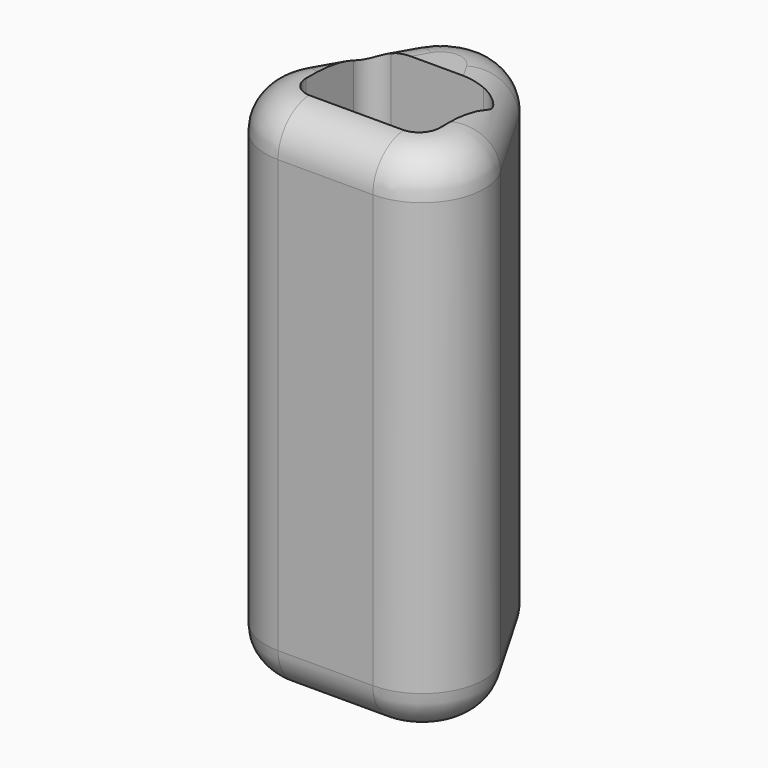
from build123d import *

# Parameters (mm, degrees)
F1_DEPTH     = 25
F2_T1_DEPTH  = 4.6076951546
F2_T3_DEPTH  = 4.6076951546
F2_T5_DEPTH  = 4.6076951546
F2_T8_ANGLE  = 120
F2_T10_ANGLE = 120
F2_T12_ANGLE = 120
F2_T14_ANGLE = 120
F2_T16_ANGLE = 120
F2_T18_ANGLE = 120


# Not quite as in the source:
# - a fillet or chamfer that OpenCascade refuses, or shapes differently, is made with other operations: its cross-section is extruded or revolved along the edge and cut away or added


with BuildPart() as f1:
    # F0 (on Top) → F1 (new body)
    with BuildSketch(Plane.XY):
        with BuildLine():
            Line((-2.3038475773, -4.3301270189), (2.3038475773, -4.3301270189))
            ThreePointArc((2.3038475773, -4.3301270189), (4.9019237886, -2.8301270189), (4.9019237886, 0.1698729811))
            Line((4.9019237886, 0.1698729811), (2.5980762114, 4.1602540378))
            ThreePointArc((2.5980762114, 4.1602540378), (0, 5.6602540378), (-2.5980762114, 4.1602540378))
            Line((-2.5980762114, 4.1602540378), (-4.9019237886, 0.1698729811))
            ThreePointArc((-4.9019237886, 0.1698729811), (-4.9019237886, -2.8301270189), (-2.3038475773, -4.3301270189))
        make_face()
        with BuildLine():
            ThreePointArc((3.25, -1.45), (2.9571067812, -2.1571067812), (2.25, -2.45))
            Line((2.25, -2.45), (-2.25, -2.45))
            ThreePointArc((-2.25, -2.45), (-2.9571067812, -2.1571067812), (-3.25, -1.45))
            Line((-3.25, -1.45), (-3.25, 1.45))
            ThreePointArc((-3.25, 1.45), (-2.9571067812, 2.1571067812), (-2.25, 2.45))
            Line((-2.25, 2.45), (2.25, 2.45))
            ThreePointArc((2.25, 2.45), (2.9571067812, 2.1571067812), (3.25, 1.45))
            Line((3.25, 1.45), (3.25, -1.45))
        make_face(mode=Mode.SUBTRACT)
    extrude(amount=F1_DEPTH)

    # F2: fillet of radius 2 on 12 edges, made by hand

    # F2_s2 → F2_t1 (cut)
    with BuildSketch(Plane(origin=(1.1519237886, -1.9951905284, 0), x_dir=(0, 0, 1), z_dir=(-0.5, 0.8660254038, 0))):
        with BuildLine():
            ThreePointArc((23, 4.3301270189), (24.4142135624, 3.7443405813), (25, 2.3301270189))
            Line((25, 2.3301270189), (25, 4.3301270189))
            Line((25, 4.3301270189), (23, 4.3301270189))
        make_face()
        with BuildLine():
            ThreePointArc((2, 4.3301270189), (0.5857864376, 3.7443405813), (0, 2.3301270189))
            Line((0, 2.3301270189), (0, 4.3301270189))
            Line((0, 4.3301270189), (2, 4.3301270189))
        make_face()
    extrude(amount=F2_T1_DEPTH, mode=Mode.SUBTRACT)

    # F2_s4 → F2_t3 (cut)
    with BuildSketch(Plane(origin=(1.1519237886, 1.9951905284, 0), x_dir=(0, 0, 1), z_dir=(-0.5, -0.8660254038, 0))):
        with BuildLine():
            ThreePointArc((23, 4.3301270189), (24.4142135624, 3.7443405813), (25, 2.3301270189))
            Line((25, 2.3301270189), (25, 4.3301270189))
            Line((25, 4.3301270189), (23, 4.3301270189))
        make_face()
        with BuildLine():
            ThreePointArc((2, 4.3301270189), (0.5857864376, 3.7443405813), (0, 2.3301270189))
            Line((0, 2.3301270189), (0, 4.3301270189))
            Line((0, 4.3301270189), (2, 4.3301270189))
        make_face()
    extrude(amount=F2_T3_DEPTH, mode=Mode.SUBTRACT)

    # F2_s6 → F2_t5 (cut)
    with BuildSketch(Plane.YZ.offset(-2.3038475773)):
        with BuildLine():
            ThreePointArc((-4.3301270189, 23), (-3.7443405813, 24.4142135624), (-2.3301270189, 25))
            Line((-2.3301270189, 25), (-4.3301270189, 25))
            Line((-4.3301270189, 25), (-4.3301270189, 23))
        make_face()
        with BuildLine():
            ThreePointArc((-4.3301270189, 2), (-3.7443405813, 0.5857864376), (-2.3301270189, 0))
            Line((-2.3301270189, 0), (-4.3301270189, 0))
            Line((-4.3301270189, 0), (-4.3301270189, 2))
        make_face()
    extrude(amount=F2_T5_DEPTH, mode=Mode.SUBTRACT)

    # F2_s7 → F2_t8 (revolve, cut)
    with BuildSketch(Plane(origin=(-1.1519237886, 1.9951905284, 0), x_dir=(0, 0, 1), z_dir=(0.5, -0.8660254038, 0))):
        with BuildLine():
            ThreePointArc((23, -4.3301270189), (24.4142135624, -3.7443405813), (25, -2.3301270189))
            Line((25, -2.3301270189), (25, -4.3301270189))
            Line((25, -4.3301270189), (23, -4.3301270189))
        make_face()
    revolve(axis=Axis((0, 2.6602540378, 25), (0, 0, 1)), revolution_arc=F2_T8_ANGLE, mode=Mode.SUBTRACT)

    # F2_s9 → F2_t10 (revolve, cut)
    with BuildSketch(Plane(origin=(-1.1519237886, -1.9951905284, 0), x_dir=(0, 0, 1), z_dir=(0.5, 0.8660254038, 0))):
        with BuildLine():
            ThreePointArc((23, -4.3301270189), (24.4142135624, -3.7443405813), (25, -2.3301270189))
            Line((25, -2.3301270189), (25, -4.3301270189))
            Line((25, -4.3301270189), (23, -4.3301270189))
        make_face()
    revolve(axis=Axis((-2.3038475773, -1.3301270189, 25), (0, 0, 1)), revolution_arc=F2_T10_ANGLE, mode=Mode.SUBTRACT)

    # F2_s11 → F2_t12 (revolve, cut)
    with BuildSketch(Plane.YZ.offset(2.3038475773)):
        with BuildLine():
            ThreePointArc((-4.3301270189, 23), (-3.7443405813, 24.4142135624), (-2.3301270189, 25))
            Line((-2.3301270189, 25), (-4.3301270189, 25))
            Line((-4.3301270189, 25), (-4.3301270189, 23))
        make_face()
    revolve(axis=Axis((2.3038475773, -1.3301270189, 25), (0, 0, 1)), revolution_arc=F2_T12_ANGLE, mode=Mode.SUBTRACT)

    # F2_s13 → F2_t14 (revolve, cut)
    with BuildSketch(Plane.YZ.offset(2.3038475773)):
        with BuildLine():
            ThreePointArc((-4.3301270189, 2), (-3.7443405813, 0.5857864376), (-2.3301270189, 0))
            Line((-2.3301270189, 0), (-4.3301270189, 0))
            Line((-4.3301270189, 0), (-4.3301270189, 2))
        make_face()
    revolve(axis=Axis((2.3038475773, -1.3301270189, 0), (0, 0, 1)), revolution_arc=F2_T14_ANGLE, mode=Mode.SUBTRACT)

    # F2_s15 → F2_t16 (revolve, cut)
    with BuildSketch(Plane(origin=(-1.1519237886, 1.9951905284, 0), x_dir=(0, 0, 1), z_dir=(0.5, -0.8660254038, 0))):
        with BuildLine():
            ThreePointArc((2, -4.3301270189), (0.5857864376, -3.7443405813), (0, -2.3301270189))
            Line((0, -2.3301270189), (0, -4.3301270189))
            Line((0, -4.3301270189), (2, -4.3301270189))
        make_face()
    revolve(axis=Axis((0, 2.6602540378, 0), (0, 0, 1)), revolution_arc=F2_T16_ANGLE, mode=Mode.SUBTRACT)

    # F2_s17 → F2_t18 (revolve, cut)
    with BuildSketch(Plane(origin=(-1.1519237886, -1.9951905284, 0), x_dir=(0, 0, 1), z_dir=(0.5, 0.8660254038, 0))):
        with BuildLine():
            ThreePointArc((2, -4.3301270189), (0.5857864376, -3.7443405813), (0, -2.3301270189))
            Line((0, -2.3301270189), (0, -4.3301270189))
            Line((0, -4.3301270189), (2, -4.3301270189))
        make_face()
    revolve(axis=Axis((-2.3038475773, -1.3301270189, 0), (0, 0, 1)), revolution_arc=F2_T18_ANGLE, mode=Mode.SUBTRACT)


solid = f1.part
